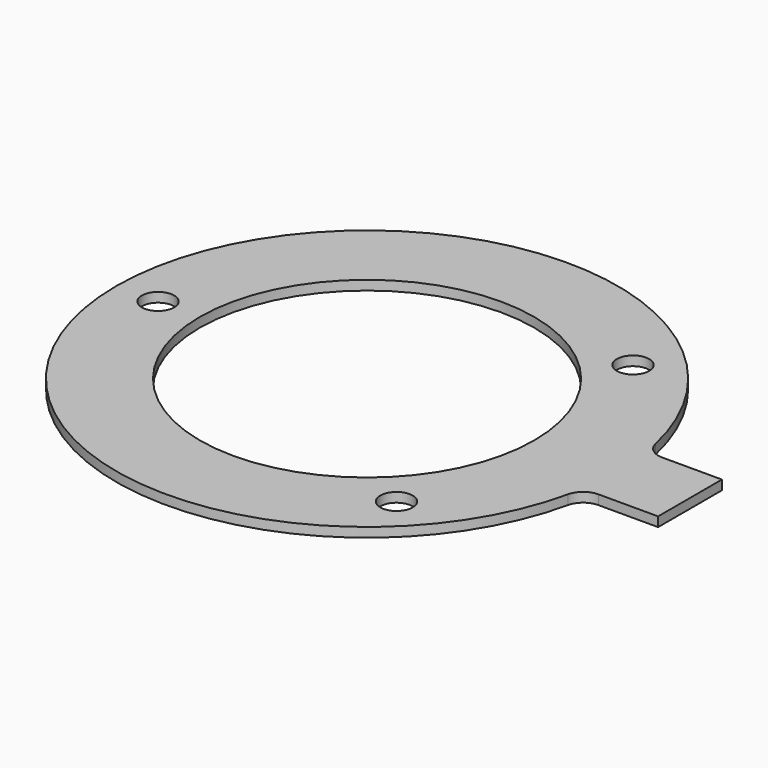
from build123d import *

# Parameters (mm, degrees)
F0_R     = 4.25
F0_R_2   = 44
F1_DEPTH = 2.5
F2_R     = 5


with BuildPart() as f1:
    # F0 (on Top) → F1 (new body)
    with BuildSketch(Plane.XY):
        with BuildLine():
            Line((85, 10.5), (65.1594198869, 10.5))
            ThreePointArc((65.1594198869, 10.5), (-66, 0), (65.1594198869, -10.5))
            Line((65.1594198869, -10.5), (85, -10.5))
            Line((85, -10.5), (85, 10.5))
        make_face()
        with Locations((38.8817437881, -38.9)):
            Circle(F0_R, mode=Mode.SUBTRACT)
        with Locations((-55, 0)):
            Circle(F0_R, mode=Mode.SUBTRACT)
        Circle(F0_R_2, mode=Mode.SUBTRACT)
        with Locations((38.8817437881, 38.9)):
            Circle(F0_R, mode=Mode.SUBTRACT)
    extrude(amount=F1_DEPTH)

    # F2
    f2_edges = [f1.edges().sort_by_distance(p)[0] for p in [
        (65.15942, 10.5, 1.25),
        (65.15942, -10.5, 1.25),
    ]]
    fillet(f2_edges, radius=F2_R)


solid = f1.part
